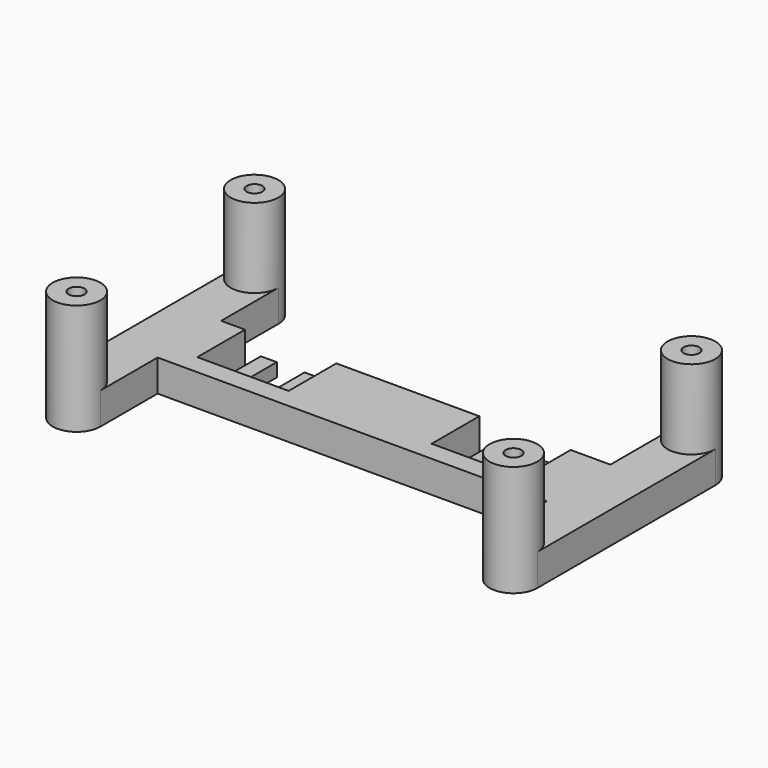
from build123d import *

# Parameters (mm, degrees)
F1_DEPTH = 4
F2_W     = 2
F2_H     = 7.5
F3_DEPTH = 1.7
F5_DEPTH = 10
F6_R     = 1
F7_DEPTH = 25


with BuildPart() as f1:
    # F0 (on Top) → F1 (new body)
    with BuildSketch(Plane.XY):
        with BuildLine():
            Line((6, 0), (55, 0))
            Line((55, 0), (55, -9))
            ThreePointArc((55, -9), (58, -12), (61, -9))
            Line((61, -9), (61, 19))
            ThreePointArc((61, 19), (58, 22), (55, 19))
            Line((55, 19), (55, 10))
            Line((55, 10), (50, 10))
            Line((50, 10), (50, 2.5))
            Line((50, 2.5), (38.5, 2.5))
            Line((38.5, 2.5), (38.5, 10))
            Line((38.5, 10), (20.5, 10))
            Line((20.5, 10), (20.5, 2.5))
            Line((20.5, 2.5), (9, 2.5))
            Line((9, 2.5), (9, 10))
            Line((9, 10), (6, 10))
            Line((6, 10), (6, 19))
            ThreePointArc((6, 19), (3, 22), (0, 19))
            Line((0, 19), (0, -9))
            ThreePointArc((0, -9), (3, -12), (6, -9))
            Line((6, -9), (6, 0))
        make_face()
    extrude(amount=F1_DEPTH)

    # F2 (on Top) → F3 (join)
    with BuildSketch(Plane.XY):
        with Locations((12, 6.25)):
            Rectangle(F2_W, F2_H)
        with Locations((17.5, 6.25)):
            Rectangle(F2_W, F2_H)
        with Locations((41.5, 6.25)):
            Rectangle(F2_W, F2_H)
        with Locations((47, 6.25)):
            Rectangle(F2_W, F2_H)
    extrude(amount=F3_DEPTH)

    # F4 (on face) → F5 (join)
    with BuildSketch(Plane.XY.offset(4)):
        with BuildLine():
            ThreePointArc((0, 19), (3, 16), (6, 19))
            ThreePointArc((6, 19), (3, 22), (0, 19))
        make_face()
        with BuildLine():
            ThreePointArc((6, -9), (3, -6), (0, -9))
            ThreePointArc((0, -9), (3, -12), (6, -9))
        make_face()
        with BuildLine():
            ThreePointArc((61, -9), (58, -6), (55, -9))
            ThreePointArc((55, -9), (58, -12), (61, -9))
        make_face()
        with BuildLine():
            ThreePointArc((55, 19), (58, 16), (61, 19))
            ThreePointArc((61, 19), (58, 22), (55, 19))
        make_face()
    extrude(amount=F5_DEPTH)

    # F6 (on face) → F7 (cut)
    with BuildSketch(Plane(origin=(0, 0, 0), x_dir=(1, 0, 0), z_dir=(0, 0, -1))):
        with Locations((3, 9)):
            Circle(F6_R)
        with Locations((58, 9)):
            Circle(F6_R)
        with Locations((58, -19)):
            Circle(F6_R)
        with Locations((3, -19)):
            Circle(F6_R)
    extrude(amount=-F7_DEPTH, mode=Mode.SUBTRACT)


solid = f1.part
